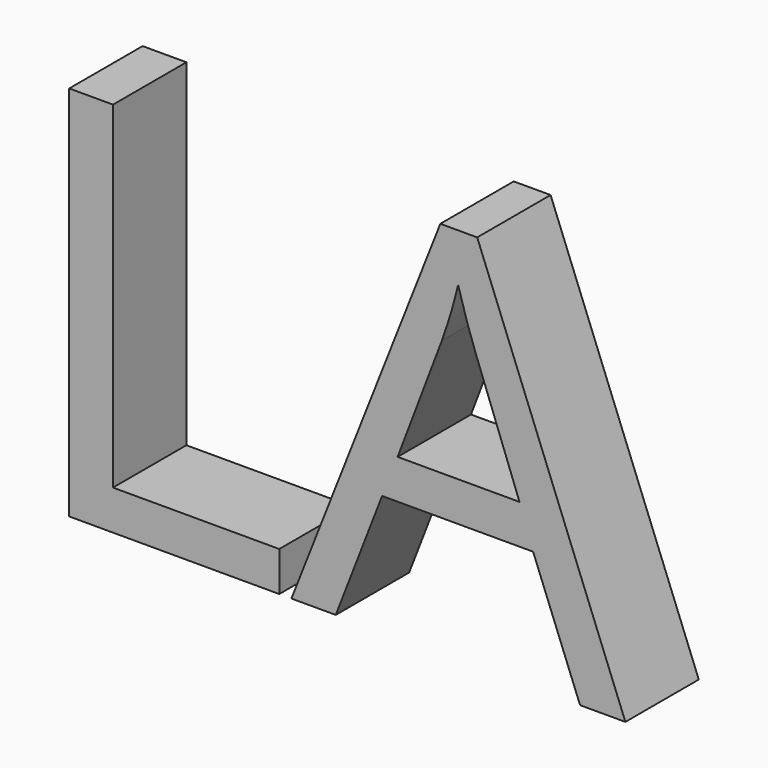
from build123d import *

# Parameters (mm, degrees)
F0_TEXT_SIZE = 71.6090357552
F1_DEPTH     = 12.446


# Not quite as in the source:
# - Text() gives the source's letters only with a copy of the font that has no kerning and outlines rounded to 1/6400 em; it was checked with that copy


with BuildPart() as f1:
    # F0 (on Front) → F1 (new body)
    with BuildSketch(Plane.XZ):
        with Locations((-43.7815545592, -18.4780433774)):
            Text('LA', F0_TEXT_SIZE, font='Open Sans', text_align=(TextAlign.LEFT, TextAlign.BOTTOM))
    extrude(amount=F1_DEPTH)


solid = f1.part
